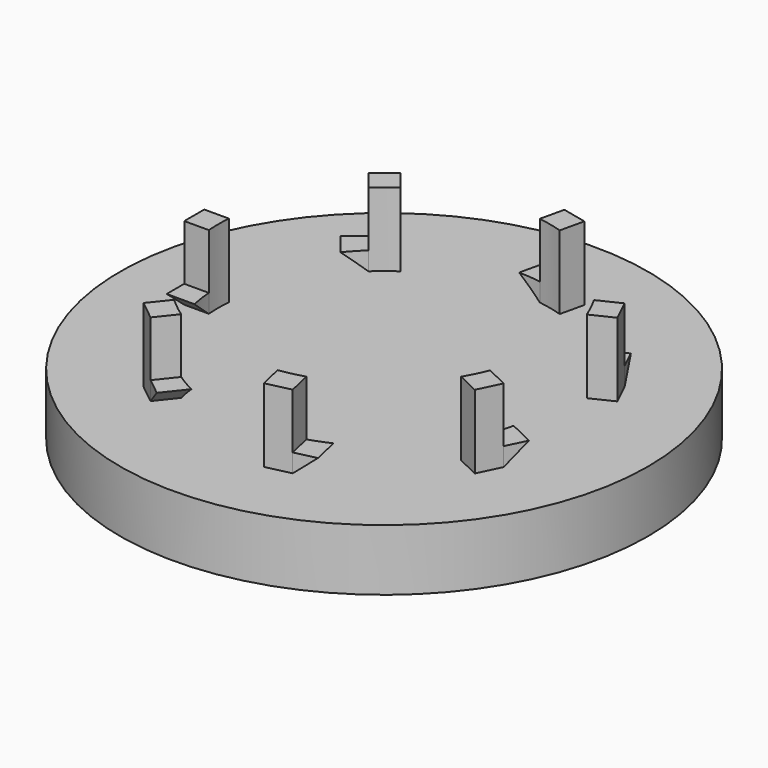
from build123d import *

# Parameters (mm, degrees)
F0_R            = 21.5
F0_R_2          = 13.5
F1_DEPTH        = 5
F3_DEPTH        = 6
F4_R            = 5.125
F5_DEPTH        = 4.5
F7_END_RADIUS   = 13.5
F7_REACH        = 39.2960714607
F7_COPIES_COUNT = 7


# Not quite as in the source:
# - a pattern or mirror of a feature is missing from the dataset's text; its kind, count and spacing are read off the source's solid


with BuildPart() as f1:
    # F0 (on Top) → F1 (new body)
    with BuildSketch(Plane.XY):
        Circle(F0_R)
        Circle(F0_R_2, mode=Mode.SUBTRACT)
        Circle(F0_R_2)
    extrude(amount=F1_DEPTH)

    # F2 (on face) → F3 (join)
    with BuildSketch(Plane.XY.offset(5)):
        with BuildLine():
            ThreePointArc((-13.4614857204, -1.0190202158), (-13.5, 0), (-13.4614857204, 1.0190202158))
            Line((-13.4614857204, 1.0190202158), (-15.4614857204, 1.0190202158))
            Line((-15.4614857204, 1.0190202158), (-15.4614857204, -1.0190202158))
            Line((-15.4614857204, -1.0190202158), (-13.4614857204, -1.0190202158))
        make_face()
        with BuildLine():
            ThreePointArc((-7.5963969786, -11.1599620494), (-8.4171123251, -10.5547250133), (-9.1898011505, -9.8892646246))
            Line((-9.1898011505, -9.8892646246), (-10.4367807542, -11.4529275895))
            Line((-10.4367807542, -11.4529275895), (-8.8433765823, -12.7236250143))
            Line((-8.8433765823, -12.7236250143), (-7.5963969786, -11.1599620494))
        make_face()
        with BuildLine():
            ThreePointArc((3.9889336264, -12.8972248381), (3.0040326084, -13.1615268145), (2.0019911235, -13.3507314984))
            Line((2.0019911235, -13.3507314984), (2.4470329914, -15.3005873227))
            Line((2.4470329914, -15.3005873227), (4.4339754943, -14.8470806625))
            Line((4.4339754943, -14.8470806625), (3.9889336264, -12.8972248381))
        make_face()
        with BuildLine():
            ThreePointArc((12.5705158512, -4.9226142683), (12.1630797167, -5.8574304781), (11.6862432483, -6.7588252486))
            Line((11.6862432483, -6.7588252486), (13.4881809841, -7.6265927268))
            Line((13.4881809841, -7.6265927268), (14.372453587, -5.7903817465))
            Line((14.372453587, -5.7903817465), (12.5705158512, -4.9226142683))
        make_face()
        with BuildLine():
            ThreePointArc((11.6862432483, 6.7588252486), (12.1630797167, 5.8574304781), (12.5705158512, 4.9226142683))
            Line((12.5705158512, 4.9226142683), (14.372453587, 5.7903817465))
            Line((14.372453587, 5.7903817465), (13.4881809841, 7.6265927268))
            Line((13.4881809841, 7.6265927268), (11.6862432483, 6.7588252486))
        make_face()
        with BuildLine():
            ThreePointArc((2.0019911235, 13.3507314984), (3.0040326084, 13.1615268145), (3.9889336264, 12.8972248381))
            Line((3.9889336264, 12.8972248381), (4.4339754943, 14.8470806625))
            Line((4.4339754943, 14.8470806625), (2.4470329914, 15.3005873227))
            Line((2.4470329914, 15.3005873227), (2.0019911235, 13.3507314984))
        make_face()
        with BuildLine():
            ThreePointArc((-9.1898011505, 9.8892646246), (-8.4171123251, 10.5547250133), (-7.5963969786, 11.1599620494))
            Line((-7.5963969786, 11.1599620494), (-8.8433765823, 12.7236250143))
            Line((-8.8433765823, 12.7236250143), (-10.4367807542, 11.4529275895))
            Line((-10.4367807542, 11.4529275895), (-9.1898011505, 9.8892646246))
        make_face()
    extrude(amount=F3_DEPTH)

    # F4 (on face) → F5 (cut)
    with BuildSketch(Plane(origin=(0, 0, 0), x_dir=(1, 0, 0), z_dir=(0, 0, -1))):
        with Locations((-14.875, 0)):
            Circle(F4_R)
        with Locations((14.875, 0)):
            Circle(F4_R)
    extrude(amount=-F5_DEPTH, mode=Mode.SUBTRACT)

    f7_end = (Plane(origin=(0, 0, 8), x_dir=(-1, 0, 0), z_dir=(0, 0, -1)) * Cylinder(F7_END_RADIUS, 202.1882593652, mode=Mode.PRIVATE)).faces().sort_by_distance((-13.5, 0, 8))[0]
    # F6 (on face) → F7 (join, up to the whole of a round face its end follows)
    with BuildSketch(Plane(origin=(-15.4614857204, 0, 0), x_dir=(0, -1, 0), z_dir=(-1, 0, 0))):
        Polygon((1.0190202158, 6.5), (1.0190202158, 5), (2.8066506047, 6.5), align=None)
    f7_long = extrude(amount=-F7_REACH, mode=Mode.PRIVATE)
    f7 = split(f7_long, bisect_by=f7_end, keep=Keep.ALL, mode=Mode.PRIVATE).solids().sort_by_distance((-15.4614857204, -1.6148970121, 6))[0]
    add(f7)

    # F7_copies: F7 ×7 about axis
    f7_copies_axis = Axis((0, 0, 0), (0, 0, 1))
    for i in range(1, F7_COPIES_COUNT):
        add(f7.rotate(f7_copies_axis, i * 360 / F7_COPIES_COUNT))


solid = f1.part
